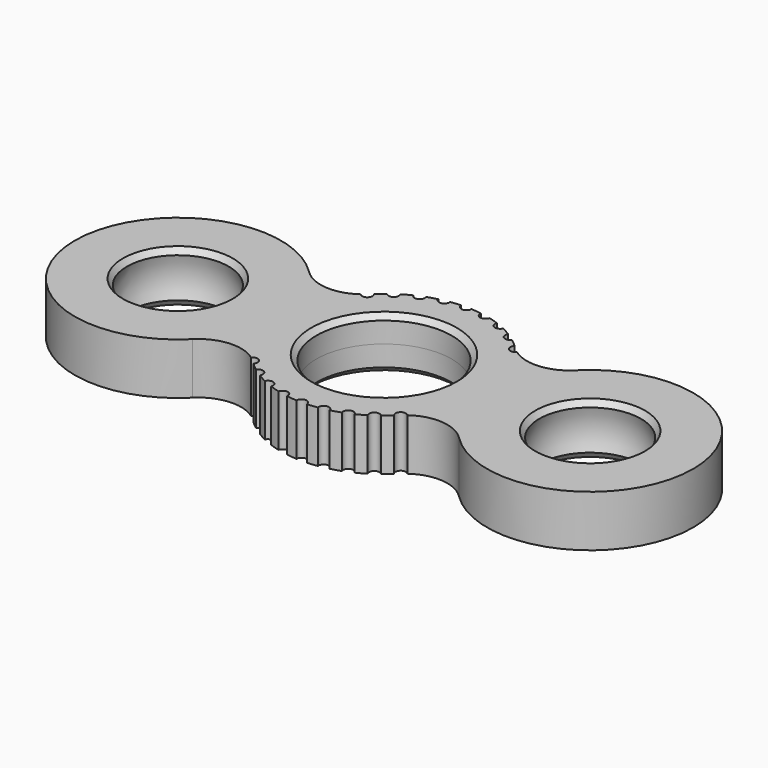
from build123d import *

# Parameters (mm, degrees)
F0_R     = 6.57
F1_DEPTH = 2.5
F2_DEPTH = 2.5
F7_SIZE  = 0.5
F8_R     = 0.5
F9_DEPTH = 25


# Not quite as in the source:
# - a fillet or chamfer that OpenCascade refuses, or shapes differently, is made with other operations: its cross-section is extruded or revolved along the edge and cut away or added


with BuildPart() as f1:
    # F0 (on Top) → F1 (new body)
    with BuildSketch(Plane.XY):
        with BuildLine():
            ThreePointArc((-12.9288643756, -7.0709999987), (-10, -5.8578081982), (-7.0711356244, -7.0709999987))
            ThreePointArc((-7.0711356244, -7.0709999987), (0, -10), (7.0711356244, -7.0709999987))
            ThreePointArc((7.0711356244, -7.0709999987), (10, -5.8578081982), (12.9288643756, -7.0709999987))
            ThreePointArc((12.9288643756, -7.0709999987), (30, 0), (12.9288643756, 7.0709999987))
            ThreePointArc((12.9288643756, 7.0709999987), (10, 5.8578081982), (7.0711356244, 7.0709999987))
            ThreePointArc((7.0711356244, 7.0709999987), (0, 10), (-7.0711356244, 7.0709999987))
            ThreePointArc((-7.0711356244, 7.0709999987), (-10, 5.8578081982), (-12.9288643756, 7.0709999987))
            ThreePointArc((-12.9288643756, 7.0709999987), (-30, 0), (-12.9288643756, -7.0709999987))
        make_face()
        Circle(F0_R, mode=Mode.SUBTRACT)
    extrude(amount=F1_DEPTH)

    # F2 (add): a face of the model
    f2_faces = [f1.faces().sort_by_distance(p)[0] for p in [
        (-10, -5.2253526661, 0),
    ]]
    extrude(f2_faces, amount=F2_DEPTH)

    # F3 (on Front) → F4 (revolve, cut)
    with BuildSketch(Plane.XZ):
        with BuildLine():
            Line((-20, -5.3), (-20, 5.3))
            ThreePointArc((-20, 5.3), (-25.3, 0), (-20, -5.3))
        make_face()
    revolve(axis=Axis((-20, 0, 0), (0, 0, -1)), mode=Mode.SUBTRACT)

    # F5 (on Front) → F6 (revolve, cut)
    with BuildSketch(Plane.XZ):
        with BuildLine():
            Line((20, 5.3), (20, -5.3))
            ThreePointArc((20, -5.3), (25.3, 0), (20, 5.3))
        make_face()
    revolve(axis=Axis((20, 0, 0), (0, 0, -1)), mode=Mode.SUBTRACT)

    # F7
    f7_edges = [f1.edges().sort_by_distance(p)[0] for p in [
        (-6.57, 0, 2.5),
        (6.57, 0, 0),
        (-6.57, 0, -2.5),
    ]]
    chamfer(f7_edges, length=F7_SIZE)

    # F8 (on face) → F9 (cut)
    with BuildSketch(Plane.XY.offset(2.5)):
        with Locations((0, 10)):
            Circle(F8_R)
        with Locations((1.9899748742, 9.8)):
            Circle(F8_R)
        with Locations((3.9003507535, 9.208)):
            Circle(F8_R)
        with Locations((5.6547126026, 8.24768)):
            Circle(F8_R)
        with Locations((7.1828859476, 6.9574528)):
            Circle(F8_R)
        with Locations((-1.9899748742, 9.8)):
            Circle(F8_R)
        with Locations((-3.9003507535, 9.208)):
            Circle(F8_R)
        with Locations((-5.6547126026, 8.24768)):
            Circle(F8_R)
        with Locations((-7.1828859476, 6.9574528)):
            Circle(F8_R)
        with Locations((7.1828859476, -6.9574528)):
            Circle(F8_R)
        with Locations((-7.1828859476, -6.9574528)):
            Circle(F8_R)
        with Locations((5.6547126026, -8.24768)):
            Circle(F8_R)
        with Locations((-5.6547126026, -8.24768)):
            Circle(F8_R)
        with Locations((-3.9003507535, -9.208)):
            Circle(F8_R)
        with Locations((1.9899748742, -9.8)):
            Circle(F8_R)
        with Locations((-1.9899748742, -9.8)):
            Circle(F8_R)
        with Locations((0, -10)):
            Circle(F8_R)
        with Locations((3.9003507535, -9.208)):
            Circle(F8_R)
    extrude(amount=-F9_DEPTH, mode=Mode.SUBTRACT)

    # F10: chamfer of 0.7 on 4 edges, made by hand

    # F10_s1 → F10_t2 (revolve, cut)
    with BuildSketch(Plane.XZ):
        with BuildLine():
            Line((25.3433302523, 2.5231214492), (24.9210794295, 1.9049078422))
            Line((24.9210794295, 1.9049078422), (24.9080386361, 1.8998149346))
            ThreePointArc((24.9080386361, 1.8998149346), (24.8038988346, 2.2055275982), (24.6609839367, 2.4933962264))
            Line((24.6609839367, 2.4933962264), (24.6733285782, 2.514))
            ThreePointArc((24.6733285782, 2.514), (25.0083294153, 2.514), (25.3433302523, 2.5371214492))
            Line((25.3433302523, 2.5371214492), (25.3433302523, 2.5231214492))
        make_face()
    revolve(axis=Axis((20, 0, 2.5), (0, 0, 1)), mode=Mode.SUBTRACT)

    # F10_s3 → F10_t4 (revolve, cut)
    with BuildSketch(Plane.XZ):
        with BuildLine():
            Line((24.9210794295, -1.9049078422), (25.3433302523, -2.5231214492))
            Line((25.3433302523, -2.5231214492), (25.3433302523, -2.5371214492))
            ThreePointArc((25.3433302523, -2.5371214492), (25.0083294153, -2.514), (24.6733285782, -2.514))
            Line((24.6733285782, -2.514), (24.6609839367, -2.4933962264))
            ThreePointArc((24.6609839367, -2.4933962264), (24.8038988346, -2.2055275982), (24.9080386361, -1.8998149346))
            Line((24.9080386361, -1.8998149346), (24.9210794295, -1.9049078422))
        make_face()
    revolve(axis=Axis((20, 0, -2.5), (0, 0, 1)), mode=Mode.SUBTRACT)

    # F10_s5 → F10_t6 (revolve, cut)
    with BuildSketch(Plane.XZ):
        with BuildLine():
            Line((-25.3433302523, 2.5231214492), (-24.9210794295, 1.9049078422))
            Line((-24.9210794295, 1.9049078422), (-24.9080386361, 1.8998149346))
            ThreePointArc((-24.9080386361, 1.8998149346), (-24.8038988346, 2.2055275982), (-24.6609839367, 2.4933962264))
            Line((-24.6609839367, 2.4933962264), (-24.6733285782, 2.514))
            ThreePointArc((-24.6733285782, 2.514), (-25.0083294153, 2.514), (-25.3433302523, 2.5371214492))
            Line((-25.3433302523, 2.5371214492), (-25.3433302523, 2.5231214492))
        make_face()
    revolve(axis=Axis((-20, 0, 2.5), (0, 0, -1)), mode=Mode.SUBTRACT)

    # F10_s7 → F10_t8 (revolve, cut)
    with BuildSketch(Plane.XZ):
        with BuildLine():
            Line((-25.3433302523, -2.5231214492), (-24.9210794295, -1.9049078422))
            Line((-24.9210794295, -1.9049078422), (-24.9080386361, -1.8998149346))
            ThreePointArc((-24.9080386361, -1.8998149346), (-24.8038988346, -2.2055275982), (-24.6609839367, -2.4933962264))
            Line((-24.6609839367, -2.4933962264), (-24.6733285782, -2.514))
            ThreePointArc((-24.6733285782, -2.514), (-25.0083294153, -2.514), (-25.3433302523, -2.5371214492))
            Line((-25.3433302523, -2.5371214492), (-25.3433302523, -2.5231214492))
        make_face()
    revolve(axis=Axis((-20, 0, -2.5), (0, 0, -1)), mode=Mode.SUBTRACT)


solid = f1.part
